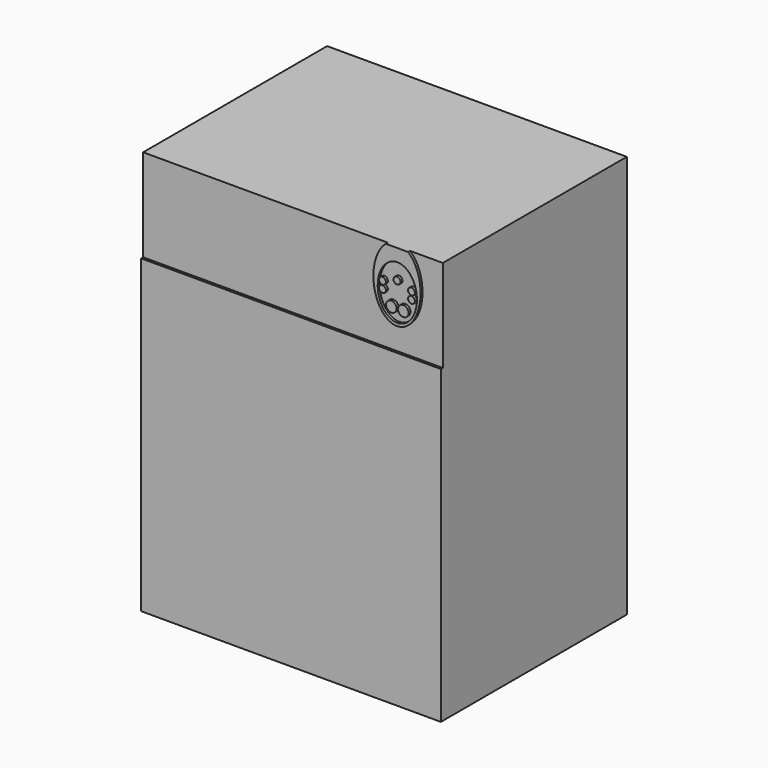
from build123d import *

# Parameters (mm, degrees)
F0_W     = 245
F0_H     = 329.5
F1_DEPTH = 190
F2_R     = 4.3236508832
F2_R_2   = 2.7917572167
F2_R_3   = 2.8466316253
F3_DEPTH = 2


# Not quite as in the source:
# - a feature names something its author has since deleted; it is built from what else it names


with BuildPart() as f1:
    # F0 (on Front) → F1 (new body)
    with BuildSketch(Plane.XZ):
        Rectangle(F0_W, F0_H)
    extrude(amount=F1_DEPTH)

    # F2 (on face) → F3 (cut)
    with BuildSketch(Plane.XZ.offset(190)):
        with BuildLine():
            add(Edge.make_bspline(
                [(86.887806654, 154.5414891056), (59.1122539749, 154.5414891056), (73.0000303144, 121.790649185), (86.887806654, 89.0398092644), (100.7755829935, 121.790649185), (114.6633593331, 154.5414891056), (86.887806654, 154.5414891056)],
                knots=[0, 0, 0, 2.0943951024, 2.0943951024, 4.1887902048, 4.1887902048, 6.2831853072, 6.2831853072, 6.2831853072], degree=2, weights=[1, 0.5, 1, 0.5, 1, 0.5, 1]))
        make_face()
        with Locations((82.0050109178, 120.968401432)):
            Circle(F2_R, mode=Mode.SUBTRACT)
        with Locations((91.7706023902, 120.968401432)):
            Circle(F2_R, mode=Mode.SUBTRACT)
        with Locations((74.7582092881, 131.2327347696)):
            Circle(F2_R_2, mode=Mode.SUBTRACT)
        with Locations((74.7582092881, 137.2206024826)):
            Circle(F2_R_2, mode=Mode.SUBTRACT)
        with Locations((86.610019207, 141.2596870214)):
            Circle(F2_R_3, mode=Mode.SUBTRACT)
        with Locations((98.4618291259, 131.2327347696)):
            Circle(F2_R_2, mode=Mode.SUBTRACT)
        with Locations((98.4618291259, 137.2206024826)):
            Circle(F2_R_2, mode=Mode.SUBTRACT)
        with BuildLine():
            add(Edge.make_bspline(
                [(77.5195354487, 164.75), (56.8220313431, 147.5523822091), (71.7160252751, 119.3755302582), (86.610019207, 91.1986783073), (101.5040131389, 119.3755302582), (116.3980070709, 147.5523822091), (95.7005029653, 164.75)],
                knots=[0.4912762616, 0.4912762616, 0.4912762616, 2.2581538563, 2.2581538563, 4.0250314509, 4.0250314509, 5.7919090456, 5.7919090456, 5.7919090456], degree=2, weights=[1, 0.6344969674, 1, 0.6344969674, 1, 0.6344969674, 1]))
            Line((77.5195354487, 164.75), (-122.5, 164.75))
            Line((-122.5, 164.75), (-122.5, 89.1870856285))
            Line((-122.5, 89.1870856285), (122.5, 89.1870856285))
            Line((122.5, 89.1870856285), (122.5, 164.75))
            Line((122.5, 164.75), (95.7005029653, 164.75))
        make_face()
    extrude(amount=-F3_DEPTH, mode=Mode.SUBTRACT)


solid = f1.part
